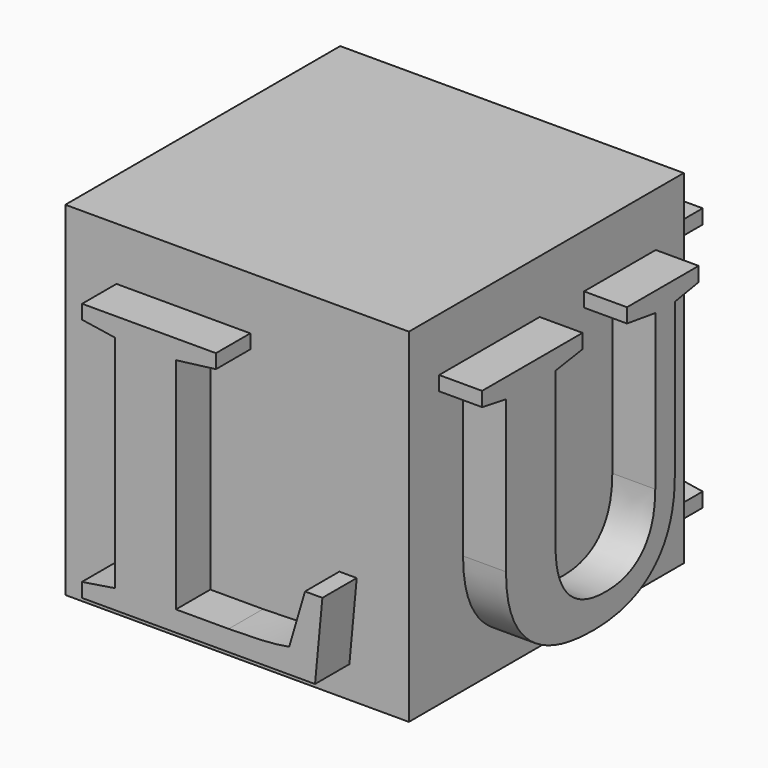
from build123d import *

# Parameters (mm, degrees)
F0_W         = 20.32
F0_H         = 20.32
F1_DEPTH     = 20.32
F2_TEXT_SIZE = 23.3947364096
F3_DEPTH     = 2.54
F4_TEXT_SIZE = 23.812500553
F5_DEPTH     = 2.54
F6_TEXT_SIZE = 23.812500553
F7_DEPTH     = 2.54
F8_TEXT_SIZE = 24.0213819779
F9_DEPTH     = 2.54


# Not quite as in the source:
# - Text() gives the source's letters only with a copy of the font that has no kerning and outlines rounded to 1/6400 em; it was checked with that copy


with BuildPart() as f1:
    # F0 (on Front) → F1 (new body)
    with BuildSketch(Plane.XZ):
        Rectangle(F0_W, F0_H)
    extrude(amount=F1_DEPTH)

    # F2 (on face) → F3 (join)
    with BuildSketch(Plane.XZ.offset(20.32)):
        with Locations((-7.5470353477, -8.2986735506)):
            Text('L', F2_TEXT_SIZE, font='Tinos', font_style=FontStyle.BOLD, text_align=(TextAlign.LEFT, TextAlign.BOTTOM))
    extrude(amount=F3_DEPTH)

    # F4 (on face) → F5 (join)
    with BuildSketch(Plane.YZ.offset(10.16)):
        with Locations((-18.6762465164, -8.5994630354)):
            Text('U', F4_TEXT_SIZE, font='Tinos', font_style=FontStyle.BOLD, text_align=(TextAlign.LEFT, TextAlign.BOTTOM))
    extrude(amount=F5_DEPTH)

    # F6 (on face) → F7 (join)
    with BuildSketch(Plane(origin=(0, 0, 0), x_dir=(-1, 0, 0), z_dir=(0, 1, 0))):
        with Locations((-9.6525618865, -8.599463501)):
            Text('K', F6_TEXT_SIZE, font='Tinos', font_style=FontStyle.BOLD, text_align=(TextAlign.LEFT, TextAlign.BOTTOM))
    extrude(amount=F7_DEPTH)

    # F8 (on face) → F9 (join)
    with BuildSketch(Plane(origin=(-10.16, 0, 0), x_dir=(0, -1, 0), z_dir=(-1, 0, 0))):
        with Locations((2.0133735026, -8.7938238394)):
            Text('E', F8_TEXT_SIZE, font='Tinos', font_style=FontStyle.BOLD, text_align=(TextAlign.LEFT, TextAlign.BOTTOM))
    extrude(amount=F9_DEPTH)


solid = f1.part
